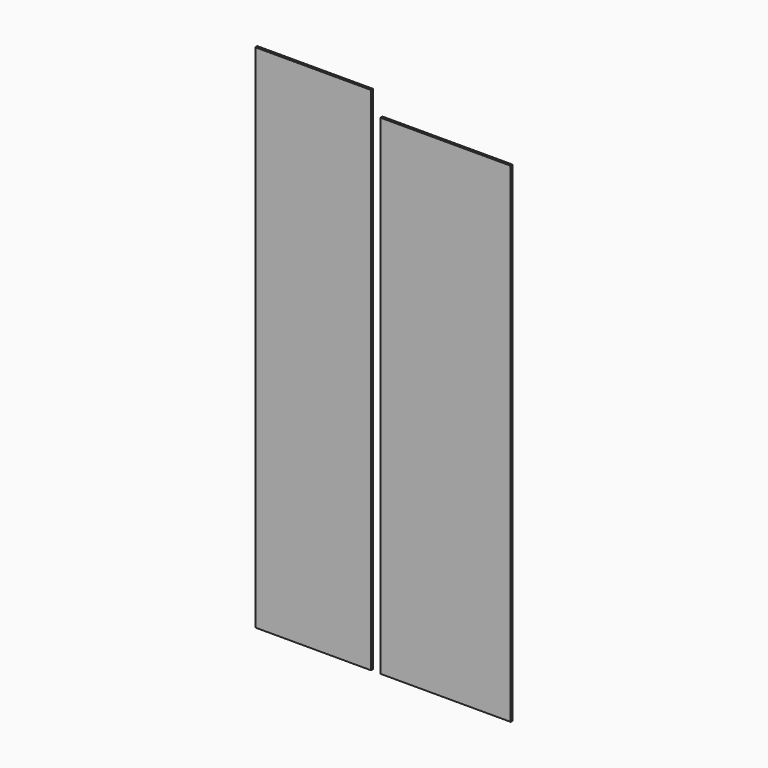
from build123d import *

# Parameters (mm, degrees)
F0_W     = 612
F0_H     = 2300
F1_DEPTH = 6
F0_W_2   = 272
F0_H_2   = 2400


with BuildPart() as f1:
    # F0 (on Front) → F1 (new body, symmetric)
    with BuildSketch(Plane.XZ):
        with Locations((294, -50)):
            Rectangle(F0_W, F0_H)
    extrude(amount=F1_DEPTH, both=True)


with BuildPart() as f1b:
    # F0 (on Front) → F1, piece 2 (new body, symmetric)
    with BuildSketch(Plane.XZ):
        with Locations((-192, 0)):
            Rectangle(F0_W_2, F0_H_2)
        with Locations((-464, 0)):
            Rectangle(F0_W_2, F0_H_2)
    extrude(amount=F1_DEPTH, both=True)


solid = Compound([f1.part, f1b.part])
